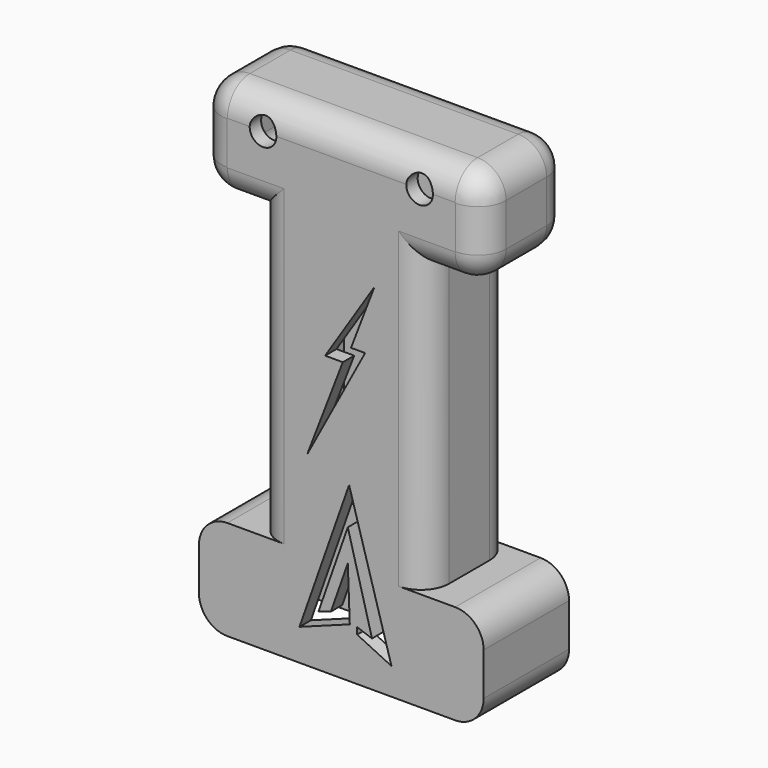
from build123d import *

# Parameters (mm, degrees)
F0_W         = 30.48
F0_H         = 50.8
F1_DEPTH     = 19.05
F2_R         = 5.08
F4_T         = -2.54
F3_R         = 2.3749
F5_DEPTH     = 45.59299
F7_DEPTH     = 16.68371
F8_DEPTH     = 25.4
F9_T1_DEPTH  = 40.64
F9_T3_DEPTH  = 7.62
F9_T5_DEPTH  = 5.08
F9_T7_DEPTH  = 5.08
F9_T10_ANGLE = 90
F9_T12_ANGLE = 90
F9_T14_ANGLE = 90
F9_T16_ANGLE = 90
F9_T18_ANGLE = 90
F9_T20_ANGLE = 90
F9_T22_ANGLE = 90
F9_T24_ANGLE = 90
F10_R        = 5


# Not quite as in the source:
# - a fillet or chamfer that OpenCascade refuses, or shapes differently, is made with other operations: its cross-section is extruded or revolved along the edge and cut away or added


with BuildPart() as f1:
    # F0 (on Front) → F1 (new body)
    with BuildSketch(Plane.XZ):
        with Locations((-8.951122936, -13.8477537125)):
            Rectangle(F0_W, F0_H)
        Polygon((6.288877064, -39.2477537125), (-24.191122936, -39.2477537125), (-34.351122936, -39.2477537125), (-34.351122936, -57.0277537125), (16.448877064, -57.0277537125), (16.448877064, -39.2477537125), align=None)
        Polygon((16.448877064, 29.3322462875), (-34.351122936, 29.3322462875), (-34.351122936, 11.5522462875), (-24.191122936, 11.5522462875), (6.288877064, 11.5522462875), (16.448877064, 11.5522462875), align=None)
    extrude(amount=F1_DEPTH)

    # F2
    f2_edges = [f1.edges().sort_by_distance(p)[0] for p in [
        (-34.351123, -9.525, 11.552246),
        (16.448877, -9.525, 11.552246),
        (16.448877, -9.525, 29.332246),
        (-34.351123, -9.525, 29.332246),
        (-34.351123, -9.525, -39.247754),
        (-34.351123, -9.525, -57.027754),
        (16.448877, -9.525, -57.027754),
        (16.448877, -9.525, -39.247754),
    ]]
    fillet(f2_edges, radius=F2_R)

    # F4: a shell. OpenCascade refuses it in one call, so the cavity is built on its own and cut out:
    # the body offset inwards by the wall thickness, plus a prism from it out through each open face.
    f4_core = offset(f1.part, amount=F4_T, kind=Kind.INTERSECTION, mode=Mode.PRIVATE)
    f4_exits = [f4_core.faces().sort_by_distance(p)[0] for p in [
        (-8.951123, -9.525, -54.487754),
    ]]
    add(f4_core, mode=Mode.SUBTRACT)
    extrude(f4_exits, amount=-F4_T, mode=Mode.SUBTRACT)

    # F3 (on face) → F5 (cut)
    with BuildSketch(Plane.XZ.offset(19.05)):
        with Locations((-22.921122936, 24.2522462875)):
            Circle(F3_R)
        with Locations((5.018877064, 24.2522462875)):
            Circle(F3_R)
    extrude(amount=-F5_DEPTH, mode=Mode.SUBTRACT)

    # F6 (on face) → F7 (cut)
    with BuildSketch(Plane.XZ.offset(19.05)):
        Polygon((-7.217857521, -4.5538423583), (-3.042159602, 6.352733355), (-11.8417982012, -7.2901686653), (-8.6815273389, -7.2901686653), (-15.0396805257, -23.8231290132), (-4.6957456507, -4.5538423583), align=None)
    extrude(amount=-F7_DEPTH, mode=Mode.SUBTRACT)

    # F6 (on face) → F8 (cut)
    with BuildSketch(Plane.XZ.offset(19.05)):
        Polygon((-7.217857521, -4.5538423583), (-3.042159602, 6.352733355), (-11.8417982012, -7.2901686653), (-8.6815273389, -7.2901686653), (-15.0396805257, -23.8231290132), (-4.6957456507, -4.5538423583), align=None)
        Polygon((-7.5618713163, -26.2167993933), (-16.4136328948, -51.3810502087), (-7.4369557778, -48.071410507), (-7.7901184559, -38.5827049613), (-10.809615066, -47.1666878623), (-13.0202344465, -47.8591975347), (-7.7901184559, -32.9299127667), (-3.4719579703, -49.0020355231), (-6.1175874434, -48.071410507), (-6.1175874434, -49.2577214361), (0, -52.201025188), align=None)
    extrude(amount=-F8_DEPTH, mode=Mode.SUBTRACT)

    # F9: fillet of radius 5 on 2 edges, made by hand

    # F9_s2 → F9_t1 (cut)
    with BuildSketch(Plane.YZ.offset(-29.271122936)):
        with BuildLine():
            ThreePointArc((-5, 29.3322462875), (-1.4644660941, 27.8677801934), (0, 24.3322462875))
            Line((0, 24.3322462875), (0, 29.3322462875))
            Line((0, 29.3322462875), (-5, 29.3322462875))
        make_face()
        with BuildLine():
            ThreePointArc((-19.05, 24.3322462875), (-17.5855339059, 27.8677801934), (-14.05, 29.3322462875))
            Line((-14.05, 29.3322462875), (-19.05, 29.3322462875))
            Line((-19.05, 29.3322462875), (-19.05, 24.3322462875))
        make_face()
    extrude(amount=F9_T1_DEPTH, mode=Mode.SUBTRACT)

    # F9_s4 → F9_t3 (cut)
    with BuildSketch(Plane.XY.offset(16.6322462875)):
        with BuildLine():
            ThreePointArc((-29.351122936, -19.05), (-32.8866568419, -17.5855339059), (-34.351122936, -14.05))
            Line((-34.351122936, -14.05), (-34.351122936, -19.05))
            Line((-34.351122936, -19.05), (-29.351122936, -19.05))
        make_face()
        with BuildLine():
            ThreePointArc((11.448877064, -19.05), (14.9844109699, -17.5855339059), (16.448877064, -14.05))
            Line((16.448877064, -14.05), (16.448877064, -19.05))
            Line((16.448877064, -19.05), (11.448877064, -19.05))
        make_face()
        with BuildLine():
            ThreePointArc((-34.351122936, -5), (-32.8866568419, -1.4644660941), (-29.351122936, 0))
            Line((-29.351122936, 0), (-34.351122936, 0))
            Line((-34.351122936, 0), (-34.351122936, -5))
        make_face()
        with BuildLine():
            ThreePointArc((16.448877064, -5), (14.9844109699, -1.4644660941), (11.448877064, 0))
            Line((11.448877064, 0), (16.448877064, 0))
            Line((16.448877064, 0), (16.448877064, -5))
        make_face()
    extrude(amount=F9_T3_DEPTH, mode=Mode.SUBTRACT)

    # F9_s6 → F9_t5 (cut)
    with BuildSketch(Plane.YZ.offset(-29.271122936)):
        with BuildLine():
            ThreePointArc((-19.05, 16.5522462875), (-17.5855339059, 13.0167123815), (-14.05, 11.5522462875))
            Line((-14.05, 11.5522462875), (-19.05, 11.5522462875))
            Line((-19.05, 11.5522462875), (-19.05, 16.5522462875))
        make_face()
        with BuildLine():
            ThreePointArc((-5, 11.5522462875), (-1.4644660941, 13.0167123815), (0, 16.5522462875))
            Line((0, 16.5522462875), (0, 11.5522462875))
            Line((0, 11.5522462875), (-5, 11.5522462875))
        make_face()
    extrude(amount=F9_T5_DEPTH, mode=Mode.SUBTRACT)

    # F9_s8 → F9_t7 (cut)
    with BuildSketch(Plane.YZ.offset(6.288877064)):
        with BuildLine():
            ThreePointArc((-19.05, 16.5522462875), (-17.5855339059, 13.0167123815), (-14.05, 11.5522462875))
            Line((-14.05, 11.5522462875), (-19.05, 11.5522462875))
            Line((-19.05, 11.5522462875), (-19.05, 16.5522462875))
        make_face()
        with BuildLine():
            ThreePointArc((-5, 11.5522462875), (-1.4644660941, 13.0167123815), (0, 16.5522462875))
            Line((0, 16.5522462875), (0, 11.5522462875))
            Line((0, 11.5522462875), (-5, 11.5522462875))
        make_face()
    extrude(amount=F9_T7_DEPTH, mode=Mode.SUBTRACT)

    # F9_s9 → F9_t10 (revolve, cut)
    with BuildSketch(Plane.XY.offset(24.2522462875)):
        with BuildLine():
            ThreePointArc((11.448877064, -19.05), (14.9844109699, -17.5855339059), (16.448877064, -14.05))
            Line((16.448877064, -14.05), (16.448877064, -19.05))
            Line((16.448877064, -19.05), (11.448877064, -19.05))
        make_face()
    revolve(axis=Axis((11.368877064, -19.05, 24.2522462875), (0, -1, 0)), revolution_arc=F9_T10_ANGLE, mode=Mode.SUBTRACT)

    # F9_s11 → F9_t12 (revolve, cut)
    with BuildSketch(Plane.YZ.offset(-29.271122936)):
        with BuildLine():
            ThreePointArc((-19.05, 24.3322462875), (-17.5855339059, 27.8677801934), (-14.05, 29.3322462875))
            Line((-14.05, 29.3322462875), (-19.05, 29.3322462875))
            Line((-19.05, 29.3322462875), (-19.05, 24.3322462875))
        make_face()
    revolve(axis=Axis((-29.271122936, -19.05, 24.2522462875), (0, -1, 0)), revolution_arc=F9_T12_ANGLE, mode=Mode.SUBTRACT)

    # F9_s13 → F9_t14 (revolve, cut)
    with BuildSketch(Plane.XY.offset(16.6322462875)):
        with BuildLine():
            ThreePointArc((-29.351122936, -19.05), (-32.8866568419, -17.5855339059), (-34.351122936, -14.05))
            Line((-34.351122936, -14.05), (-34.351122936, -19.05))
            Line((-34.351122936, -19.05), (-29.351122936, -19.05))
        make_face()
    revolve(axis=Axis((-29.271122936, -19.05, 16.6322462875), (0, -1, 0)), revolution_arc=F9_T14_ANGLE, mode=Mode.SUBTRACT)

    # F9_s15 → F9_t16 (revolve, cut)
    with BuildSketch(Plane.YZ.offset(11.368877064)):
        with BuildLine():
            ThreePointArc((-19.05, 16.5522462875), (-17.5855339059, 13.0167123815), (-14.05, 11.5522462875))
            Line((-14.05, 11.5522462875), (-19.05, 11.5522462875))
            Line((-19.05, 11.5522462875), (-19.05, 16.5522462875))
        make_face()
    revolve(axis=Axis((11.368877064, -19.05, 16.6322462875), (0, -1, 0)), revolution_arc=F9_T16_ANGLE, mode=Mode.SUBTRACT)

    # F9_s17 → F9_t18 (revolve, cut)
    with BuildSketch(Plane.XY.offset(24.2522462875)):
        with BuildLine():
            ThreePointArc((16.448877064, -5), (14.9844109699, -1.4644660941), (11.448877064, 0))
            Line((11.448877064, 0), (16.448877064, 0))
            Line((16.448877064, 0), (16.448877064, -5))
        make_face()
    revolve(axis=Axis((11.368877064, 0, 24.2522462875), (0, -1, 0)), revolution_arc=F9_T18_ANGLE, mode=Mode.SUBTRACT)

    # F9_s19 → F9_t20 (revolve, cut)
    with BuildSketch(Plane.YZ.offset(-29.271122936)):
        with BuildLine():
            ThreePointArc((-5, 29.3322462875), (-1.4644660941, 27.8677801934), (0, 24.3322462875))
            Line((0, 24.3322462875), (0, 29.3322462875))
            Line((0, 29.3322462875), (-5, 29.3322462875))
        make_face()
    revolve(axis=Axis((-29.271122936, 0, 24.2522462875), (0, -1, 0)), revolution_arc=F9_T20_ANGLE, mode=Mode.SUBTRACT)

    # F9_s21 → F9_t22 (revolve, cut)
    with BuildSketch(Plane.XY.offset(16.6322462875)):
        with BuildLine():
            ThreePointArc((-34.351122936, -5), (-32.8866568419, -1.4644660941), (-29.351122936, 0))
            Line((-29.351122936, 0), (-34.351122936, 0))
            Line((-34.351122936, 0), (-34.351122936, -5))
        make_face()
    revolve(axis=Axis((-29.271122936, 0, 16.6322462875), (0, -1, 0)), revolution_arc=F9_T22_ANGLE, mode=Mode.SUBTRACT)

    # F9_s23 → F9_t24 (revolve, cut)
    with BuildSketch(Plane.YZ.offset(11.368877064)):
        with BuildLine():
            ThreePointArc((-5, 11.5522462875), (-1.4644660941, 13.0167123815), (0, 16.5522462875))
            Line((0, 16.5522462875), (0, 11.5522462875))
            Line((0, 11.5522462875), (-5, 11.5522462875))
        make_face()
    revolve(axis=Axis((11.368877064, 0, 16.6322462875), (0, -1, 0)), revolution_arc=F9_T24_ANGLE, mode=Mode.SUBTRACT)

    # F10
    f10_edges = [f1.edges().sort_by_distance(p)[0] for p in [
        (6.288877, 0, -11.347754),
        (6.288877, -19.05, -11.347754),
        (-24.191123, 0, -11.347754),
        (-24.191123, -19.05, -11.347754),
    ]]
    fillet(f10_edges, radius=F10_R)


solid = f1.part
